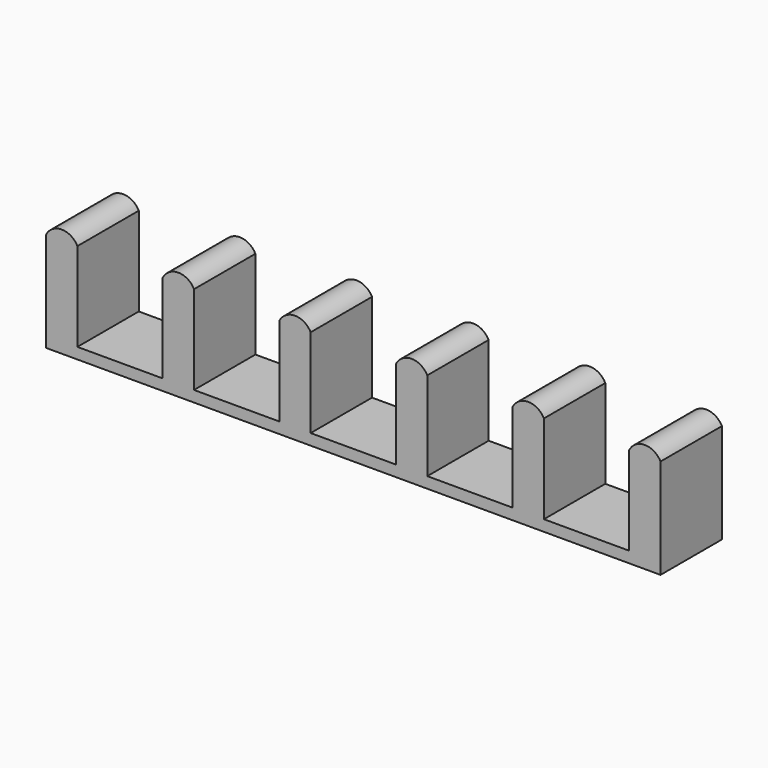
from build123d import *

# Parameters (mm, degrees)
F1_DEPTH = 25


# Not quite as in the source:
# - a feature names something its author has since deleted; it is built from what else it names


with BuildPart() as f1:
    # F0 (on Front) → F1 (new body)
    with BuildSketch(Plane.XZ):
        with BuildLine():
            Line((-38.1111986935, 28.9119444788), (-38.1111986935, 0))
            Line((-38.1111986935, 0), (-27.9069803655, 0))
            Line((-27.9069803655, 0), (-27.9069803655, 28.9119444788))
            ThreePointArc((-27.9069803655, 28.9119444788), (-33.0090895295, 32.0041291416), (-38.1111986935, 28.9119444788))
        make_face()
        with BuildLine():
            Line((-0.1111986935, 28.9119444788), (-0.1111986935, 0))
            Line((-0.1111986935, 0), (10.0930196345, 0))
            Line((10.0930196345, 0), (10.0930196345, 28.9119444788))
            ThreePointArc((10.0930196345, 28.9119444788), (4.9909104705, 32.0041291416), (-0.1111986935, 28.9119444788))
        make_face()
        with BuildLine():
            Line((37.8888013065, 28.9119444788), (37.8888013065, 0))
            Line((37.8888013065, 0), (48.0930196345, 0))
            Line((48.0930196345, 0), (48.0930196345, 28.9119444788))
            ThreePointArc((48.0930196345, 28.9119444788), (42.9909104705, 32.0041291416), (37.8888013065, 28.9119444788))
        make_face()
        with BuildLine():
            Line((75.8888013065, 28.9119444788), (75.8888013065, 0))
            Line((75.8888013065, 0), (86.0930196345, 0))
            Line((86.0930196345, 0), (86.0930196345, 28.9119444788))
            ThreePointArc((86.0930196345, 28.9119444788), (80.9909104705, 32.0041291416), (75.8888013065, 28.9119444788))
        make_face()
        with BuildLine():
            Line((113.8888013065, 0), (124.0930196345, 0))
            Line((124.0930196345, 0), (124.0930196345, 28.9119444788))
            ThreePointArc((124.0930196345, 28.9119444788), (118.9909104705, 32.0041291416), (113.8888013065, 28.9119444788))
            Line((113.8888013065, 28.9119444788), (113.8888013065, 0))
        make_face()
        with BuildLine():
            Line((151.8888013065, 0), (162.0930196345, 0))
            Line((162.0930196345, 0), (162.0930196345, 28.9119444788))
            ThreePointArc((162.0930196345, 28.9119444788), (156.9909104705, 32.0041291416), (151.8888013065, 28.9119444788))
            Line((151.8888013065, 28.9119444788), (151.8888013065, 0))
        make_face()
        Polygon((-27.9069803655, 0), (-38.1111986935, 0), (-38.1111986935, -3.615781432), (162.0930196345, -3.615781432), (162.0930196345, 0), (151.8888013065, 0), (146.6320851445, 0), (131.5820539594, 0), (124.0930196345, 0), (113.8888013065, 0), (108.6320851445, 0), (93.5820539594, 0), (86.0930196345, 0), (75.8888013065, 0), (70.6320851445, 0), (55.5820539594, 0), (48.0930196345, 0), (37.8888013065, 0), (32.6320851445, 0), (10.0930196345, 0), (-0.1111986935, 0), (-5.3679148555, 0), align=None)
    extrude(amount=F1_DEPTH)


solid = f1.part
